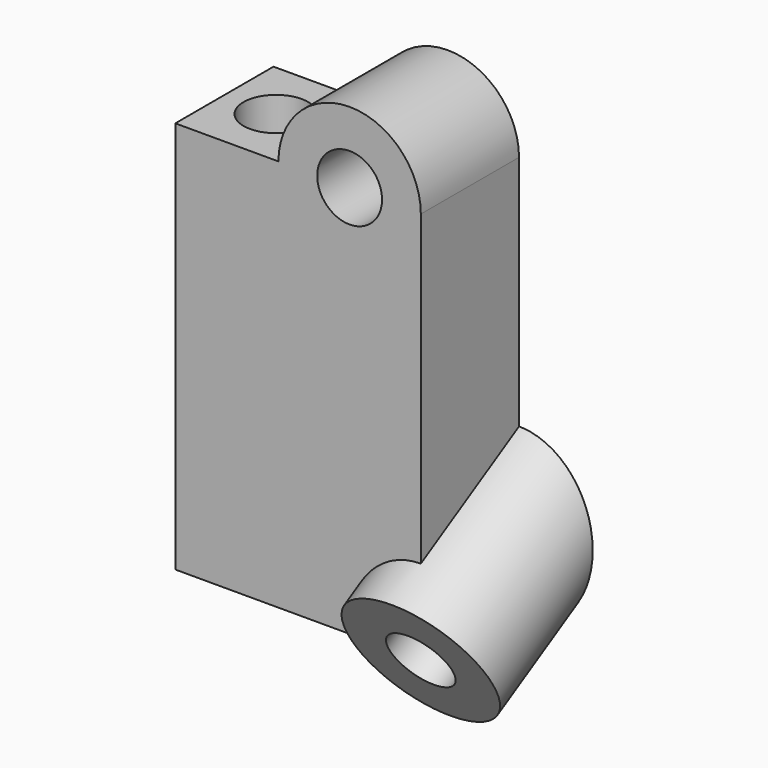
from build123d import *

# Parameters (mm, degrees)
F1_DEPTH        = 25
F3_D            = 13.2
F3_CBORE_D      = 19.25
F3_CBORE_DEPTH  = 0
F4_W            = 24.2927655578
F4_H            = 50
F5_DEPTH        = 60
F7_D            = 13.2
F7_CBORE_D      = 19.25
F7_CBORE_DEPTH  = 0
F9_R            = 15
F10_DEPTH       = 52
F12_D           = 13.2
F12_CBORE_D     = 19.25
F12_CBORE_DEPTH = 0
F13_W           = 29.7532882541
F13_H           = 56.5460538492
F14_DEPTH       = 50


with BuildPart() as f1:
    # F0 (on Front) → F1 (new body)
    with BuildSketch(Plane.XZ):
        with BuildLine():
            Line((-25, -40), (25, -40))
            Line((25, -40), (25, 40))
            ThreePointArc((25, 40), (10.5, 25.5), (-4, 40))
            Line((-4, 40), (-25, 40))
            Line((-25, 40), (-25, -40))
        make_face()
        with BuildLine():
            ThreePointArc((-4, 40), (10.5, 25.5), (25, 40))
            Line((25, 40), (-4, 40))
        make_face()
        with BuildLine():
            Line((-4, 40), (25, 40))
            ThreePointArc((25, 40), (10.5, 54.5), (-4, 40))
        make_face()
    extrude(amount=F1_DEPTH)

    # F3 (through all)
    with Locations(Plane(origin=(0, 0, 0), x_dir=(-1, 0, 0), z_dir=(0, 1, 0))):
        with Locations((-10.5, 40)):
            CounterBoreHole(F3_D / 2, F3_CBORE_D / 2, F3_CBORE_DEPTH)

    # F4 (on Right) → F5 (cut)
    with BuildSketch(Plane.YZ):
        with Locations((-37.1463827789, -15)):
            Rectangle(F4_W, F4_H)
    extrude(amount=F5_DEPTH, mode=Mode.SUBTRACT)

    # F7 (through all)
    with Locations(Plane.XY.offset(40)):
        with Locations((-14.5, -12.5)):
            CounterBoreHole(F7_D / 2, F7_CBORE_D / 2, F7_CBORE_DEPTH)

    # F9 (on face) → F10 (join)
    with BuildSketch(Plane(origin=(0, -36.0705080757, -20.8253175473), x_dir=(-1, 0, 0), z_dir=(0, 0.8660254038, 0.5))):
        with Locations((-25, -22.1410161514)):
            Circle(F9_R)
    extrude(amount=F10_DEPTH)

    # F12 (through all)
    with Locations(Plane(origin=(0, -36.0705080757, -20.8253175473), x_dir=(1, 0, 0), z_dir=(0, -0.8660254038, -0.5))):
        with Locations((25, -22.1410161514)):
            CounterBoreHole(F12_D / 2, F12_CBORE_D / 2, F12_CBORE_DEPTH)

    # F13 (on Right) → F14 (cut)
    with BuildSketch(Plane.YZ):
        with Locations((14.8766441271, -15.394736547)):
            Rectangle(F13_W, F13_H)
    extrude(amount=F14_DEPTH, mode=Mode.SUBTRACT)


solid = f1.part
